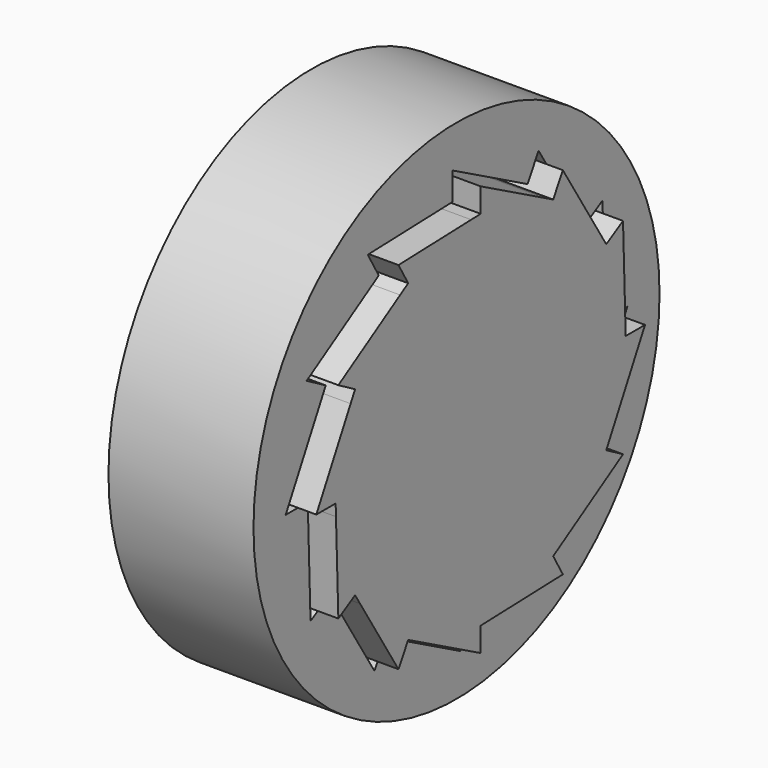
from build123d import *

# Parameters (mm, degrees)
F1_DEPTH      = 6
F0_R          = 10.5
F2_DEPTH      = 5
F2_DEPTH_BACK = 1


with BuildPart() as f1:
    # F0 (on Right) → F1 (new body)
    with BuildSketch(Plane.YZ):
        with BuildLine():
            Line((8.5, 0), (7.5, 0))
            ThreePointArc((7.5, 0), (7.3039386076, -1.7036668737), (6.7260051156, -3.3182608675))
            Line((6.7260051156, -3.3182608675), (8.5, 0))
        make_face()
        with BuildLine():
            ThreePointArc((6.7260051156, -3.3182608675), (7.3039386076, -1.7036668737), (7.5, 0))
            Line((7.5, 0), (7.4840217299, 0.4893043502))
            ThreePointArc((7.4840217299, 0.4893043502), (7.1772298187, 2.1765505116), (6.4951905284, 3.75))
            Line((6.4951905284, 3.75), (6.2367007655, 4.1657608623))
            ThreePointArc((6.2367007655, 4.1657608623), (5.127388096, 5.473562945), (3.75, 6.4951905284))
            Line((3.75, 6.4951905284), (3.3182608675, 6.7260051156))
            ThreePointArc((3.3182608675, 6.7260051156), (1.7036668737, 7.3039386076), (0, 7.5))
            Line((0, 7.5), (-0.4893043502, 7.4840217299))
            ThreePointArc((-0.4893043502, 7.4840217299), (-2.1765505116, 7.1772298187), (-3.75, 6.4951905284))
            Line((-3.75, 6.4951905284), (-4.1657608623, 6.2367007655))
            ThreePointArc((-4.1657608623, 6.2367007655), (-5.473562945, 5.127388096), (-6.4951905284, 3.75))
            Line((-6.4951905284, 3.75), (-6.7260051156, 3.3182608675))
            ThreePointArc((-6.7260051156, 3.3182608675), (-7.3039386076, 1.7036668737), (-7.5, 0))
            Line((-7.5, 0), (-7.4840217299, -0.4893043502))
            ThreePointArc((-7.4840217299, -0.4893043502), (-7.1772298187, -2.1765505116), (-6.4951905284, -3.75))
            Line((-6.4951905284, -3.75), (-6.2367007655, -4.1657608623))
            ThreePointArc((-6.2367007655, -4.1657608623), (-5.127388096, -5.473562945), (-3.75, -6.4951905284))
            Line((-3.75, -6.4951905284), (-3.3182608675, -6.7260051156))
            ThreePointArc((-3.3182608675, -6.7260051156), (-1.7036668737, -7.3039386076), (0, -7.5))
            Line((0, -7.5), (0.4893043502, -7.4840217299))
            ThreePointArc((0.4893043502, -7.4840217299), (2.1765505116, -7.1772298187), (3.75, -6.4951905284))
            Line((3.75, -6.4951905284), (4.1657608623, -6.2367007655))
            ThreePointArc((4.1657608623, -6.2367007655), (5.473562945, -5.127388096), (6.4951905284, -3.75))
            Line((6.4951905284, -3.75), (6.7260051156, -3.3182608675))
        make_face()
        with BuildLine():
            ThreePointArc((6.4951905284, 3.75), (7.1772298187, 2.1765505116), (7.4840217299, 0.4893043502))
            Line((7.4840217299, 0.4893043502), (7.3612159322, 4.25))
            Line((7.3612159322, 4.25), (6.4951905284, 3.75))
        make_face()
        with BuildLine():
            Line((7.3612159322, -4.25), (6.4951905284, -3.75))
            ThreePointArc((6.4951905284, -3.75), (5.473562945, -5.127388096), (4.1657608623, -6.2367007655))
            Line((4.1657608623, -6.2367007655), (7.3612159322, -4.25))
        make_face()
        with BuildLine():
            ThreePointArc((3.75, 6.4951905284), (5.127388096, 5.473562945), (6.2367007655, 4.1657608623))
            Line((6.2367007655, 4.1657608623), (4.25, 7.3612159322))
            Line((4.25, 7.3612159322), (3.75, 6.4951905284))
        make_face()
        with BuildLine():
            Line((4.25, -7.3612159322), (3.75, -6.4951905284))
            ThreePointArc((3.75, -6.4951905284), (2.1765505116, -7.1772298187), (0.4893043502, -7.4840217299))
            Line((0.4893043502, -7.4840217299), (4.25, -7.3612159322))
        make_face()
        with BuildLine():
            ThreePointArc((0, 7.5), (1.7036668737, 7.3039386076), (3.3182608675, 6.7260051156))
            Line((3.3182608675, 6.7260051156), (0, 8.5))
            Line((0, 8.5), (0, 7.5))
        make_face()
        with BuildLine():
            Line((0, -8.5), (0, -7.5))
            ThreePointArc((0, -7.5), (-1.7036668737, -7.3039386076), (-3.3182608675, -6.7260051156))
            Line((-3.3182608675, -6.7260051156), (0, -8.5))
        make_face()
        with BuildLine():
            ThreePointArc((-3.75, 6.4951905284), (-2.1765505116, 7.1772298187), (-0.4893043502, 7.4840217299))
            Line((-0.4893043502, 7.4840217299), (-4.25, 7.3612159322))
            Line((-4.25, 7.3612159322), (-3.75, 6.4951905284))
        make_face()
        with BuildLine():
            Line((-4.25, -7.3612159322), (-3.75, -6.4951905284))
            ThreePointArc((-3.75, -6.4951905284), (-5.127388096, -5.473562945), (-6.2367007655, -4.1657608623))
            Line((-6.2367007655, -4.1657608623), (-4.25, -7.3612159322))
        make_face()
        with BuildLine():
            ThreePointArc((-6.4951905284, 3.75), (-5.473562945, 5.127388096), (-4.1657608623, 6.2367007655))
            Line((-4.1657608623, 6.2367007655), (-7.3612159322, 4.25))
            Line((-7.3612159322, 4.25), (-6.4951905284, 3.75))
        make_face()
        with BuildLine():
            Line((-7.3612159322, -4.25), (-6.4951905284, -3.75))
            ThreePointArc((-6.4951905284, -3.75), (-7.1772298187, -2.1765505116), (-7.4840217299, -0.4893043502))
            Line((-7.4840217299, -0.4893043502), (-7.3612159322, -4.25))
        make_face()
        with BuildLine():
            ThreePointArc((-7.5, 0), (-7.3039386076, 1.7036668737), (-6.7260051156, 3.3182608675))
            Line((-6.7260051156, 3.3182608675), (-8.5, 0))
            Line((-8.5, 0), (-7.5, 0))
        make_face()
    extrude(amount=F1_DEPTH)


with BuildPart() as f2:
    # F0 (on Right) → F2 (new body, two sides)
    with BuildSketch(Plane.YZ) as f2_sk:
        Circle(F0_R)
        Polygon((-3.6735826839, -6.7628320185), (-4.2436502465, -7.7502180007), (-6.5628319364, -4.0199929876), (-7.5502179186, -4.5900605502), (-7.6935756715, -0.2000000821), (-8.8337107967, -0.2000000821), (-6.7628320185, 3.6735826839), (-7.7502180007, 4.2436502465), (-4.0199929876, 6.5628319364), (-4.5900605502, 7.5502179186), (-0.2000000821, 7.6935756715), (-0.2000000821, 8.8337107967), (3.6735826839, 6.7628320185), (4.2436502465, 7.7502180007), (6.5628319364, 4.0199929876), (7.5502179186, 4.5900605502), (7.6935756715, 0.2000000821), (8.8337107967, 0.2000000821), (6.7628320185, -3.6735826839), (7.7502180007, -4.2436502465), (4.0199929876, -6.5628319364), (4.5900605502, -7.5502179186), (0.2000000821, -7.6935756715), (0.2000000821, -8.8337107967), align=None, mode=Mode.SUBTRACT)
    extrude(amount=F2_DEPTH)
    extrude(f2_sk.sketch, amount=-F2_DEPTH_BACK)


solid = Compound([f1.part, f2.part])
